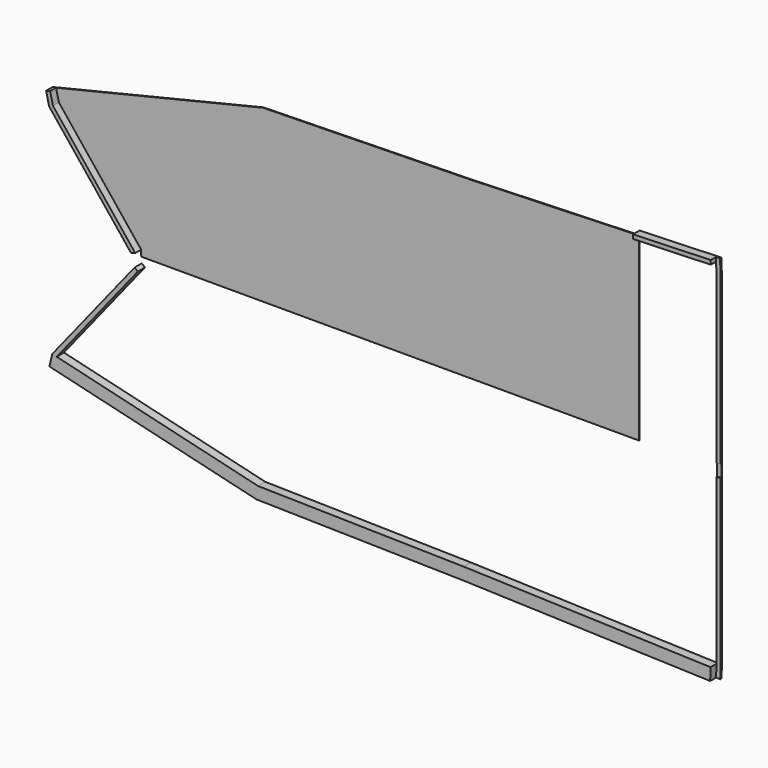
from build123d import *

# Parameters (mm, degrees)
F1_DEPTH = 0.2
F2_DEPTH = 2
F3_DEPTH = 2.2
F6_DEPTH = 0.4


# Not quite as in the source:
# - a feature of the source that left no trace in its solid (it failed there, or was rolled back) is left out
# - a feature names something its author has since deleted; it is built from what else it names


with BuildPart() as f1:
    # F0 (on Front) → F1 (new body)
    with BuildSketch(Plane.XZ):
        Polygon((-31.8378226987, 37), (-81.8378226987, 25), (-61.8378226987, 0), (-61.813899618, -1.4998092166), (59.1621773013, -1.4998092166), (59.1621773013, 39.3666666667), (18.1621773013, 38), align=None)
        Polygon((-82.5379415561, 27.9171619059), (-81.8378226987, 25), (-31.8378226987, 37), (18.1621773013, 38), (59.1621773013, 39.3666666667), (59.1621773013, 42.3683328706), (18.0822075051, 40.9990005441), (-32.2223249338, 39.9929098953), align=None)
    extrude(amount=F1_DEPTH)

    # F0 (on Front) → F2 (join)
    with BuildSketch(Plane.XZ):
        Polygon((-61.8378226987, 0), (-81.8378226987, 25), (-82.5379415561, 27.9171619059), (-83.5103288581, 27.6837889535), (-82.7581217792, 24.5495927912), (-62.8322434414, -0.357755131), align=None)
        Polygon((59.1621773013, 43.3688882719), (59.1621773013, 42.3683328706), (78.0622328106, 42.9983347209), (78.0289179803, 43.9977796279), align=None)
    extrude(amount=F2_DEPTH)



with BuildPart() as f1b:
    # F0 (on Front) → F1, piece 2 (new body)
    with BuildSketch(Plane.XZ):
        Polygon((79.1621773013, 0), (78.1621773013, 0), (78.1621773013, -1.4998092166), (78.1621773013, -2.9996184332), (79.1621773013, -2.9996184332), (79.1621773013, -1.4998092166), align=None)
    extrude(amount=F1_DEPTH)


with BuildPart() as f3:
    # F0 (on Front) → F3 (new body)
    with BuildSketch(Plane.XZ):
        Polygon((-80.7634729945, -28.2574623622), (-81.8378226987, -27.9996184332), (-82.5379415561, -30.9167803391), (-32.2223249338, -42.9925283285), (18.0822075051, -43.9986189773), (78.0622328106, -45.9979531541), (78.1621773013, -42.9996184332), (18.1621773013, -40.9996184332), (-31.8378226987, -39.9996184332), align=None)
        Polygon((-61.0569538893, -3.6243134808), (-61.8378226987, -2.9996184332), (-81.8378226987, -27.9996184332), (-80.7634729945, -28.2574623622), align=None)
    extrude(amount=F3_DEPTH)


with BuildPart() as f1_1:
    add(f1.part)

    add(f1b.part)  # F6 merges F1b

    add(f3.part)  # F6 merges F3
    # F0 (on Front) → F6 (join)
    with BuildSketch(Plane.XZ):
        Polygon((78.0289179803, 43.9977796279), (78.0622328106, 42.9983347209), (78.1621773013, 40), (78.1621773013, 0), (79.1621773013, 0), (79.1621773013, 40.0166620396), (79.0616777176, 43.0316495512), (79.0283628873, 44.0310944581), align=None)
        Polygon((78.1621773013, -42.9996184332), (78.0622328106, -45.9979531541), (79.0616777176, -46.0312679844), (79.1621773013, -43.0162804728), (79.1621773013, -2.9996184332), (78.1621773013, -2.9996184332), align=None)
    extrude(amount=F6_DEPTH)


solid = f1_1.part
